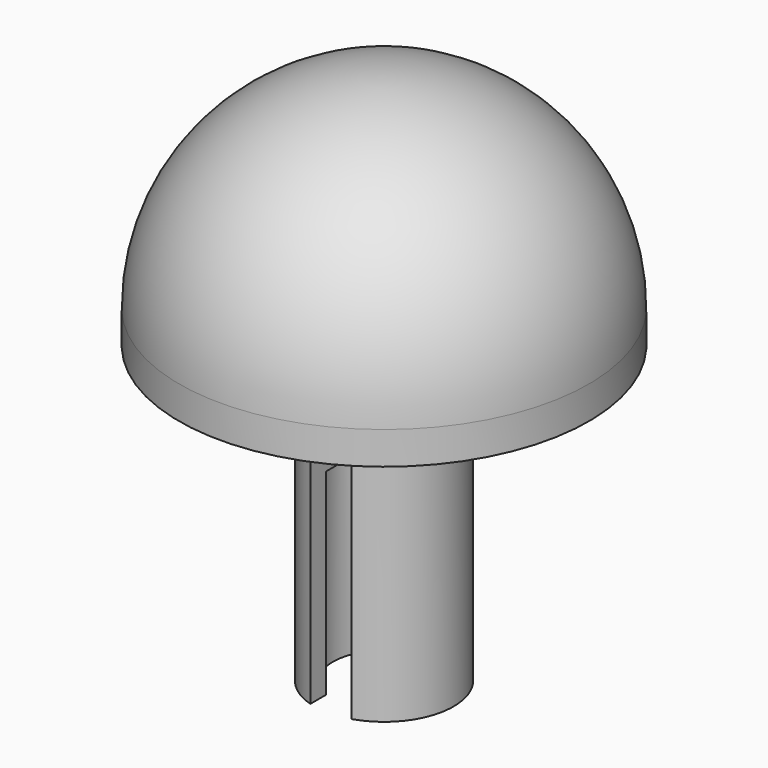
from build123d import *
from build123d import SkipClean  # not in build123d's __all__

# Parameters (mm, degrees)
F2_R      = 1.25
F3_DEPTH  = 8.001
F5_R      = 1.25
F5_R_2    = 0.9
F6_DEPTH  = 3.2
F7_W      = 1
F7_H      = 4
F8_DEPTH  = 8
F9_R      = 0.9
F10_DEPTH = 2


with BuildPart() as f1:
    # F0 (on Right) → F1 (revolve)
    with BuildSketch(Plane.YZ):
        with BuildLine():
            Line((5, -0.8), (5, 0))
            ThreePointArc((5, 0), (3.5355339059, 3.5355339059), (0, 5))
            Line((0, 5), (0, -8))
            Line((0, -8), (1.7, -8))
            Line((1.7, -8), (1.7, 0))
            Line((1.7, 0), (4.6, 0))
            Line((4.6, 0), (4.6, -0.8))
            Line((4.6, -0.8), (5, -0.8))
        make_face()
    revolve(axis=Axis((0, 0, -1.5), (0, 0, -1)))

    # F2 (on Top) → F3 (cut, through all)
    with BuildSketch(Plane.XY):
        Circle(F2_R)
    extrude(amount=-F3_DEPTH, mode=Mode.SUBTRACT)

    # F5 (on face) → F6 (join)
    with BuildSketch(Plane(origin=(0, 0, 0), x_dir=(1, 0, 0), z_dir=(0, 0, -1))):
        Circle(F5_R)
        Circle(F5_R_2, mode=Mode.SUBTRACT)
    extrude(amount=F6_DEPTH)

    # F7 (on face) → F8 (cut, through all)
    with BuildSketch(Plane(origin=(0, 0, -8), x_dir=(1, 0, 0), z_dir=(0, 0, -1))):
        Rectangle(F7_W, F7_H)
    extrude(amount=-F8_DEPTH, mode=Mode.SUBTRACT)

    # F9 (on face) → F10 (cut)
    with BuildSketch(Plane(origin=(0, 0, 0), x_dir=(1, 0, 0), z_dir=(0, 0, -1))):
        Circle(F9_R)
    with SkipClean():  # cleaning this boolean's faces spoils the solid; the shape is the same uncleaned
        extrude(amount=-F10_DEPTH, mode=Mode.SUBTRACT)


solid = f1.part
